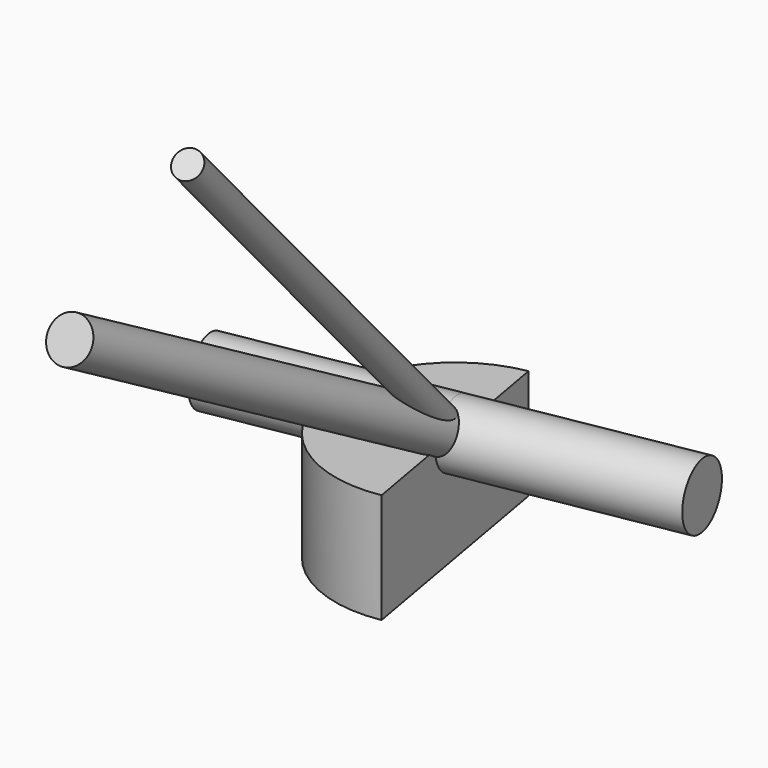
from build123d import *

# Parameters (mm, degrees)
F5_DEPTH      = 12.7
F8_R          = 3.7324399965
F9_DEPTH      = 25.4
F9_DEPTH_BACK = 25.4


with BuildPart() as f3:
    # F0 (on Right) → F3 (revolve)
    with BuildSketch(Plane.YZ):
        Polygon((-54.3816796127, 34.3302167309), (-55.6516796127, 32.1305122053), (0, 0), (0.6109335276, 2.5802167309), align=None)
    revolve(axis=Axis((0, -33.598147265, 19.3978993677), (0, -0.8660254038, 0.5)))


with BuildPart() as f5:
    # F4 (on line) → F5 (new body)
    with BuildSketch(Plane(origin=(0, 0, 0), x_dir=(1, 0, 0), z_dir=(0, 0, -1))):
        with BuildLine():
            Line((0, 0), (2.4004124433, 13.6134154491))
            ThreePointArc((2.4004124433, 13.6134154491), (-13.6134154491, 2.4004124433), (-2.4004124433, -13.6134154491))
            Line((-2.4004124433, -13.6134154491), (0, 0))
        make_face()
    extrude(amount=F5_DEPTH)

    # F8 (on face) → F9 (join, two sides)
    with BuildSketch(Plane(origin=(0, 0, 0), x_dir=(-0.1736481777, 0.984807753, 0), z_dir=(0.984807753, 0.1736481777, 0))) as f9_sk:
        Circle(F8_R)
    extrude(amount=F9_DEPTH)
    extrude(f9_sk.sketch, amount=-F9_DEPTH_BACK)


with BuildPart() as f7:
    # F6 (on face) → F7 (revolve)
    with BuildSketch(Plane(origin=(0, 0, 0), x_dir=(-0.1736481777, 0.984807753, 0), z_dir=(0.984807753, 0.1736481777, 0))):
        Polygon((2.4517506192, -4.7163042091), (0, 0), (-50.2975093123, 50.2975093123), (-51.4297861072, 49.1652325173), align=None)
    revolve(axis=Axis((5.3802521718, -30.5129263268, 30.9836373987), (0.122787804, -0.6963642403, 0.7071067812)))


solid = Compound([f3.part, f5.part, f7.part])
